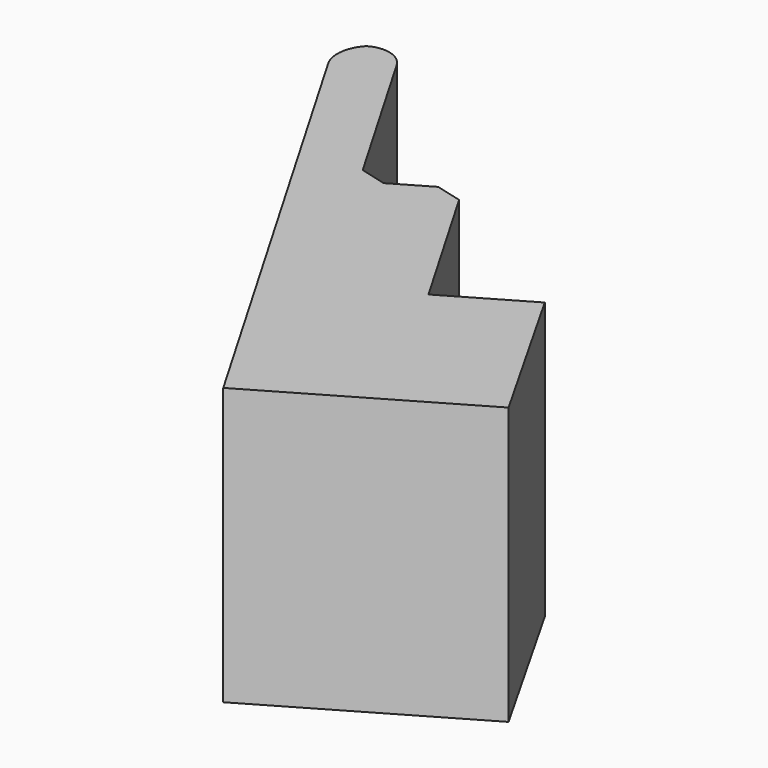
from build123d import *

# Parameters (mm, degrees)
F1_DEPTH    = 72.644
F2_R        = 7.3585229381
F3_SIZE     = 5.08
F4_SIZE     = 5.08
F5_T1_DEPTH = 116.8137644874


# Not quite as in the source:
# - a fillet or chamfer that OpenCascade refuses, or shapes differently, is made with other operations: its cross-section is extruded or revolved along the edge and cut away or added


with BuildPart() as f1:
    # F0 (on Top) → F1 (new body)
    with BuildSketch(Plane.XY):
        Polygon((-24.6386431996, 69.7602594984), (-36.737293005, 62.7278536558), (40.861338377, -70.7739219069), (91.9838476343, -41.0586860274), (68.6385333538, 0), (47.8052062724, -12.1094844007), (23.9140867359, 28.9931332809), (5.3346716929, 18.1937474815), align=None)
    extrude(amount=F1_DEPTH)

    # F2
    f2_edges = [f1.edges().sort_by_distance(p)[0] for p in [
        (-24.638643, 69.760259, 36.322),
    ]]
    fillet(f2_edges, radius=F2_R)

    # F3
    f3_edges = [f1.edges().sort_by_distance(p)[0] for p in [
        (5.334672, 18.193747, 36.322),
    ]]
    chamfer(f3_edges, length=F3_SIZE)

    # F4
    f4_edges = [f1.edges().sort_by_distance(p)[0] for p in [
        (23.914087, 28.993133, 36.322),
    ]]
    chamfer(f4_edges, length=F4_SIZE)

    # F5: fillet of radius 9.1981536726 on 1 edges, made by hand

    # F5_s2 → F5_t1 (cut)
    with BuildSketch(Plane.XY.offset(-22.0848822437)):
        with BuildLine():
            ThreePointArc((-31.0005259261, 66.0623806462), (-33.480123973, 60.7928785055), (-32.2979662711, 55.0903735776))
            Line((-32.2979662711, 55.0903735776), (-36.737293005, 62.7278536558))
            Line((-36.737293005, 62.7278536558), (-31.0005259261, 66.0623806462))
        make_face()
    extrude(amount=F5_T1_DEPTH, mode=Mode.SUBTRACT)


solid = f1.part
